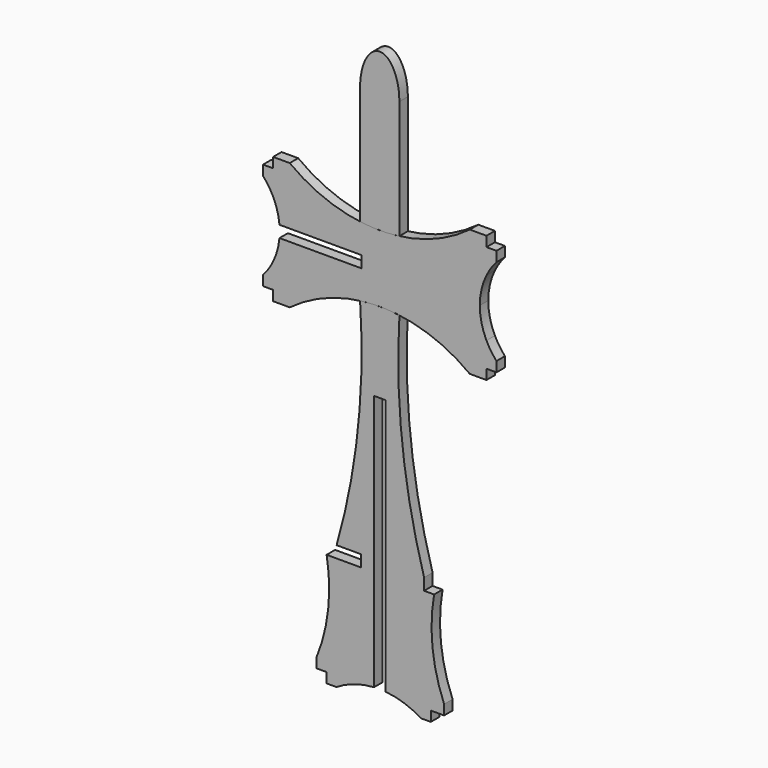
from build123d import *

# Parameters (mm, degrees)
F1_DEPTH = 3.175
F3_DEPTH = 3.175
F4_W     = 7.2773662827
F4_H     = 3.5
F5_DEPTH = 3.1760001


# Not quite as in the source:
# - a length typed as a fraction of an inch, garbled in the dataset ("3 / 203.2 mm" for 3/8 in), is restored


with BuildPart() as f1:
    # F0 (on Front) → F1 (new body)
    with BuildSketch(Plane.XZ):
        with BuildLine():
            Line((32, -16.05), (35, -16.05))
            Line((35, -16.05), (35, -13.05))
            ThreePointArc((35, -13.05), (33.3469639854, -10.9330653905), (32, -8.6093553766))
            Line((32, -8.6093553766), (32, -16.05))
        make_face()
        with BuildLine():
            ThreePointArc((32, 8.6093553766), (33.3469639854, 10.9330653905), (35, 13.05))
            Line((35, 13.05), (35, 16.05))
            Line((35, 16.05), (32, 16.05))
            Line((32, 16.05), (32, 8.6093553766))
        make_face()
        with BuildLine():
            Line((-35, -16.05), (-32, -16.05))
            Line((-32, -16.05), (-32, -8.6093553766))
            ThreePointArc((-32, -8.6093553766), (-33.3469639854, -10.9330653905), (-35, -13.05))
            Line((-35, -13.05), (-35, -16.05))
        make_face()
        with BuildLine():
            ThreePointArc((-35, 13.05), (-33.3469639854, 10.9330653905), (-32, 8.6093553766))
            Line((-32, 8.6093553766), (-32, 16.05))
            Line((-32, 16.05), (-35, 16.05))
            Line((-35, 16.05), (-35, 13.05))
        make_face()
        with BuildLine():
            Line((27, -19.05), (32, -19.05))
            Line((32, -19.05), (32, -16.05))
            Line((32, -16.05), (32, -8.6093553766))
            ThreePointArc((32, -8.6093553766), (30.5065696236, -4.4193042439), (30, 0))
            Line((30, 0), (-5.5, 0))
            Line((-5.5, 0), (-5.5, -1.75))
            Line((-5.5, -1.75), (-30.0785620254, -1.75))
            ThreePointArc((-30.0785620254, -1.75), (-30.7239047108, -5.268020684), (-32, -8.6093553766))
            Line((-32, -8.6093553766), (-32, -16.05))
            Line((-32, -16.05), (-32, -19.05))
            Line((-32, -19.05), (-27, -19.05))
            ThreePointArc((-27, -19.05), (0, -10.05), (27, -19.05))
        make_face()
        with BuildLine():
            ThreePointArc((30, 0), (30.5065696236, 4.4193042439), (32, 8.6093553766))
            Line((32, 8.6093553766), (32, 16.05))
            Line((32, 16.05), (32, 19.05))
            Line((32, 19.05), (27, 19.05))
            ThreePointArc((27, 19.05), (0, 10.05), (-27, 19.05))
            Line((-27, 19.05), (-32, 19.05))
            Line((-32, 19.05), (-32, 16.05))
            Line((-32, 16.05), (-32, 8.6093553766))
            ThreePointArc((-32, 8.6093553766), (-30.7239047108, 5.268020684), (-30.0785620254, 1.75))
            Line((-30.0785620254, 1.75), (-5.5, 1.75))
            Line((-5.5, 1.75), (-5.5, 0))
            Line((-5.5, 0), (30, 0))
        make_face()
    extrude(amount=F1_DEPTH)


with BuildPart() as f3:
    # F2 (on face) → F3 (new body)
    with BuildSketch(Plane.XZ.offset(3.175)):
        with BuildLine():
            add(Edge.make_bspline(
                [(5.9, 45.9891505916), (5.9, 57.2641204958), (0, 57.2641204958), (-5.9, 57.2641204958), (-5.9, 45.9891505916)],
                knots=[1.5707963268, 1.5707963268, 1.5707963268, 3.1415926536, 3.1415926536, 4.7123889804, 4.7123889804, 4.7123889804], degree=2, weights=[1, 0.7071067812, 1, 0.7071067812, 1]))
            Line((-5.9, 45.9891505916), (5.9, 45.9891505916))
        make_face()
        with BuildLine():
            Line((-5.9, 45.9891505916), (-5.9, 10.4384544092))
            Line((-5.9, 10.4384544092), (5.9, 10.4384544092))
            Line((5.9, 10.4384544092), (5.9, 45.9891505916))
            add(Edge.make_bspline(
                [(0, 34.7141806875), (5.9, 34.7141806875), (5.9, 45.9891505916)],
                knots=[0, 0, 0, 1.5707963268, 1.5707963268, 1.5707963268], degree=2, weights=[1, 0.7071067812, 1]))
            add(Edge.make_bspline(
                [(-5.9, 45.9891505916), (-5.9, 34.7141806875), (0, 34.7141806875)],
                knots=[4.7123889804, 4.7123889804, 4.7123889804, 6.2831853072, 6.2831853072, 6.2831853072], degree=2, weights=[1, 0.7071067812, 1]))
        make_face()
        with BuildLine():
            Line((5.9, 45.9891505916), (-5.9, 45.9891505916))
            add(Edge.make_bspline(
                [(-5.9, 45.9891505916), (-5.9, 34.7141806875), (0, 34.7141806875)],
                knots=[4.7123889804, 4.7123889804, 4.7123889804, 6.2831853072, 6.2831853072, 6.2831853072], degree=2, weights=[1, 0.7071067812, 1]))
            add(Edge.make_bspline(
                [(0, 34.7141806875), (5.9, 34.7141806875), (5.9, 45.9891505916)],
                knots=[0, 0, 0, 1.5707963268, 1.5707963268, 1.5707963268], degree=2, weights=[1, 0.7071067812, 1]))
        make_face()
        with BuildLine():
            ThreePointArc((13.2956086248, -77.2701255913), (6.7462265041, -44.1698462786), (5.9, -10.4384544092))
            Line((5.9, -10.4384544092), (-5.9, -10.4384544092))
            ThreePointArc((-5.9, -10.4384544092), (-6.5162024945, -44.1596635216), (-12.9346875995, -77.2701255913))
            Line((-12.9346875995, -77.2701255913), (13.2956086248, -77.2701255913))
        make_face()
        with BuildLine():
            Line((13.2956086248, -80.7701255913), (13.2956086248, -77.2701255913))
            Line((13.2956086248, -77.2701255913), (-12.9346875995, -77.2701255913))
            Line((-12.9346875995, -77.2701255913), (-12.9346875995, -80.7701255913))
            Line((-12.9346875995, -80.7701255913), (-15.9346875995, -80.7701255913))
            ThreePointArc((-15.9346875995, -80.7701255913), (-15.4658906298, -94.9642033946), (-18.9346875995, -108.7358795042))
            Line((-18.9346875995, -108.7358795042), (-18.9346875995, -111.7358795042))
            Line((-18.9346875995, -111.7358795042), (-15.9900602624, -111.7358795042))
            Line((-15.9900602624, -111.7358795042), (-15.9900602624, -114.7358795042))
            Line((-15.9900602624, -114.7358795042), (-12.9900602624, -114.7358795042))
            ThreePointArc((-12.9900602624, -114.7358795042), (-0.3376854584, -111.0977054943), (12.3146893457, -114.7358795042))
            Line((12.3146893457, -114.7358795042), (15.3146893457, -114.7358795042))
            Line((15.3146893457, -114.7358795042), (15.3146893457, -111.7358795042))
            Line((15.3146893457, -111.7358795042), (19.2956086248, -111.7358795042))
            Line((19.2956086248, -111.7358795042), (19.2956086248, -108.7358795042))
            ThreePointArc((19.2956086248, -108.7358795042), (15.814653799, -94.9655076172), (16.2956086248, -80.7701255913))
            Line((16.2956086248, -80.7701255913), (13.2956086248, -80.7701255913))
        make_face()
        with BuildLine():
            Line((5.9, 10.4384544092), (-5.9, 10.4384544092))
            ThreePointArc((-5.9, 10.4384544092), (0, 10.05), (5.9, 10.4384544092))
        make_face()
        with BuildLine():
            Line((-5.9, -10.4384544092), (5.9, -10.4384544092))
            ThreePointArc((5.9, -10.4384544092), (0, -10.05), (-5.9, -10.4384544092))
        make_face()
    extrude(amount=-F3_DEPTH)

    # F4 (on face) → F5 (cut, through all)
    with BuildSketch(Plane.XZ.offset(3.175)):
        with BuildLine():
            Line((-1.75, -34.1893706199), (-1.75, -111.1396121123))
            ThreePointArc((-1.75, -111.1396121123), (0.0009152594, -111.1001122679), (1.75, -111.1893706199))
            Line((1.75, -111.1893706199), (1.75, -34.1893706199))
            Line((1.75, -34.1893706199), (-1.75, -34.1893706199))
        make_face()
        with Locations((-9.2960044582, -79.0201255913)):
            Rectangle(F4_W, F4_H)
    extrude(amount=-F5_DEPTH, mode=Mode.SUBTRACT)


solid = Compound([f1.part, f3.part])
